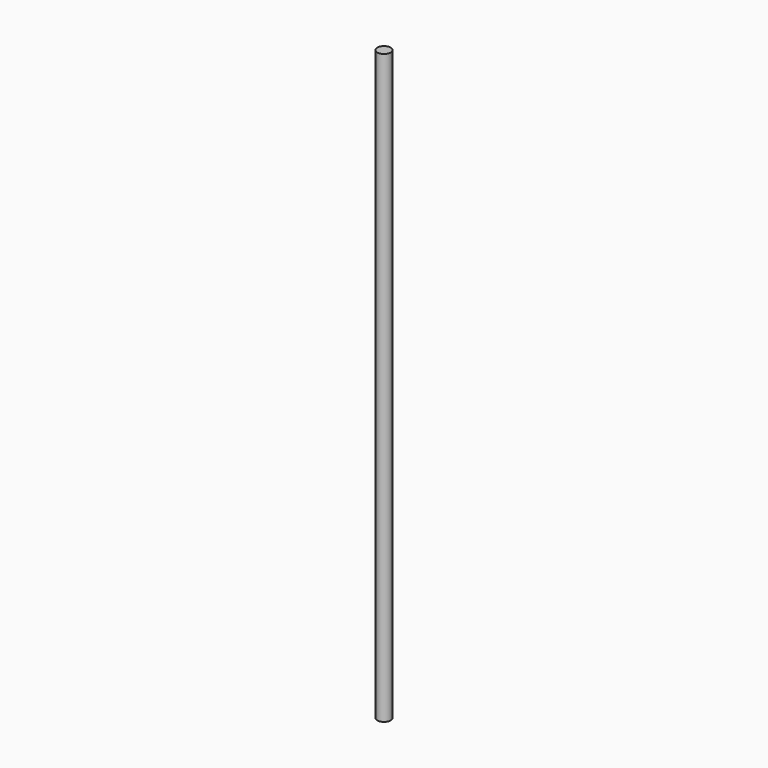
from build123d import *

# Parameters (mm, degrees)
F0_R     = 6
F0_R_2   = 5
F1_DEPTH = 525
F2_DEPTH = 404
F3_SIZE  = 0.5
F4_DEPTH = 414


with BuildPart() as f1:
    # F0 (on Top) → F1 (new body)
    with BuildSketch(Plane.XY):
        Circle(F0_R)
        Circle(F0_R_2, mode=Mode.SUBTRACT)
        Circle(F0_R_2)
    extrude(amount=F1_DEPTH)


with BuildPart() as f2:
    # F0 (on Top) → F2 (new body)
    with BuildSketch(Plane.XY):
        Circle(F0_R_2)
    extrude(amount=F2_DEPTH)

    # F3
    f3_edges = [f2.edges().sort_by_distance(p)[0] for p in [
        (-5, 0, 0),
        (-5, 0, 404),
    ]]
    chamfer(f3_edges, length=F3_SIZE)


with BuildPart() as f4:
    # F0 (on Top) → F4 (new body)
    with BuildSketch(Plane.XY):
        Circle(F0_R_2)
    extrude(amount=F4_DEPTH)


solid = Compound([f1.part, f2.part, f4.part])
